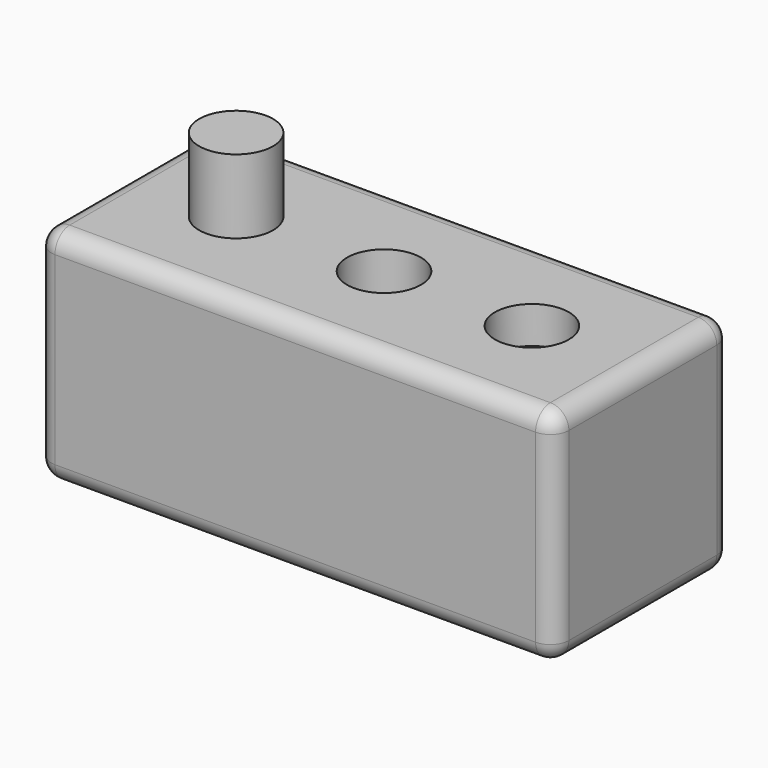
from build123d import *

# Parameters (mm, degrees)
F0_W          = 140
F0_H          = 60
F1_DEPTH      = 60
F2_R          = 10
F5_DEPTH      = 20
F4_R          = 10
F6_DEPTH      = 71.6
F3_R          = 10
F7_DEPTH      = 10
F8_R          = 5
F9_T1_DEPTH   = 165
F9_T3_DEPTH   = 67.5
F9_S7_W       = 5
F9_S7_H       = 5
F9_T8_DEPTH   = 5
F10_T1_DEPTH  = 50
F10_T3_DEPTH  = 67.5
F10_S7_W      = 5
F10_S7_H      = 5
F10_T8_DEPTH  = 5
F10_T12_ANGLE = 89.9999999974
F11_T1_DEPTH  = 147.5
F11_T3_DEPTH  = 50
F11_S7_W      = 5
F11_S7_H      = 5
F11_T8_DEPTH  = 5
F11_T12_ANGLE = 89.9999999974
F12_T1_DEPTH  = 50
F12_T3_DEPTH  = 50
F12_S7_W      = 5
F12_S7_H      = 5
F12_T8_DEPTH  = 5
F12_S13_W     = 5
F12_S13_H     = 5
F12_T14_DEPTH = 5
F12_T18_ANGLE = 89.9999999974


# Not quite as in the source:
# - a fillet or chamfer that OpenCascade refuses, or shapes differently, is made with other operations: its cross-section is extruded or revolved along the edge and cut away or added


with BuildPart() as f1:
    # F0 (on Top) → F1 (new body)
    with BuildSketch(Plane.XY):
        Rectangle(F0_W, F0_H)
    extrude(amount=F1_DEPTH)

    # F2 (on face) → F5 (join)
    with BuildSketch(Plane.XY.offset(60)):
        with Locations((-40, 0)):
            Circle(F2_R)
    extrude(amount=F5_DEPTH)

    # F4 (on face) → F6 (cut)
    with BuildSketch(Plane.XY.offset(60)):
        Circle(F4_R)
    extrude(amount=-F6_DEPTH, mode=Mode.SUBTRACT)

    # F3 (on face) → F7 (cut)
    with BuildSketch(Plane.XY.offset(60)):
        with Locations((40, 0)):
            Circle(F3_R)
    extrude(amount=-F7_DEPTH, mode=Mode.SUBTRACT)

    # F8
    f8_edges = [f1.edges().sort_by_distance(p)[0] for p in [
        (0, 30, 60),
        (-70, 0, 60),
        (0, -30, 60),
        (70, 0, 60),
    ]]
    fillet(f8_edges, radius=F8_R)

    # F9: fillet of radius 5 on 2 edges, made by hand

    # F9_s2 → F9_t1 (cut)
    with BuildSketch(Plane.YZ.offset(-82.5)):
        with BuildLine():
            ThreePointArc((-30, 5), (-28.5355339059, 1.4644660941), (-25, 0))
            Line((-25, 0), (-30, 0))
            Line((-30, 0), (-30, 5))
        make_face()
    extrude(amount=F9_T1_DEPTH, mode=Mode.SUBTRACT)

    # F9_s4 → F9_t3 (cut)
    with BuildSketch(Plane.XY.offset(-12.5)):
        with BuildLine():
            ThreePointArc((65, -30), (68.5355339059, -28.5355339059), (70, -25))
            Line((70, -25), (70, -30))
            Line((70, -30), (65, -30))
        make_face()
    extrude(amount=F9_T3_DEPTH, mode=Mode.SUBTRACT)


with BuildPart() as f9_tool6:
    # F9_s7 → F9_t8 (new body)
    with BuildSketch(Plane.XZ.offset(25)):
        with Locations((67.5, 57.5)):
            Rectangle(F9_S7_W, F9_S7_H)
    extrude(amount=F9_T8_DEPTH)

    # F9_s9 → F9_t10 (revolve, cut)
    with BuildSketch(Plane(origin=(65, -25, 55), x_dir=(-0.7071067812, 0, -0.7071067812), z_dir=(-0.7071067812, 0, 0.7071067812))):
        with BuildLine():
            ThreePointArc((0, -5), (5, 0), (0, 5))
            Line((0, 5), (0, -5))
        make_face()
    revolve(axis=Axis((65, -25, 55), (0, -1, 0)), mode=Mode.SUBTRACT)


with BuildPart() as f1_1:
    add(f1.part)

    # F9_t5: cut F9_tool6
    add(f9_tool6.part, mode=Mode.SUBTRACT)

    # F10: fillet of radius 5 on 1 edges, made by hand

    # F10_s2 → F10_t1 (cut)
    with BuildSketch(Plane.XY.offset(5)):
        with BuildLine():
            ThreePointArc((-65, -30), (-68.5355339059, -28.5355339059), (-70, -25))
            Line((-70, -25), (-70, -30))
            Line((-70, -30), (-65, -30))
        make_face()
    extrude(amount=F10_T1_DEPTH, mode=Mode.SUBTRACT)

    # F10_s4 → F10_t3 (cut)
    with BuildSketch(Plane.XZ.offset(-42.5)):
        with BuildLine():
            ThreePointArc((-70, 5), (-68.5355339059, 1.4644660941), (-65, 0))
            Line((-65, 0), (-70, 0))
            Line((-70, 0), (-70, 5))
        make_face()
    extrude(amount=F10_T3_DEPTH, mode=Mode.SUBTRACT)


with BuildPart() as f10_tool6:
    # F10_s7 → F10_t8 (new body)
    with BuildSketch(Plane.XZ.offset(25)):
        with Locations((-67.5, 57.5)):
            Rectangle(F10_S7_W, F10_S7_H)
    extrude(amount=F10_T8_DEPTH)

    # F10_s9 → F10_t10 (revolve, cut)
    with BuildSketch(Plane(origin=(-65, -25, 55), x_dir=(0.7071067812, 0, -0.7071067812), z_dir=(-0.7071067812, 0, -0.7071067812))):
        with BuildLine():
            ThreePointArc((0, -5), (5, 0), (0, 5))
            Line((0, 5), (0, -5))
        make_face()
    revolve(axis=Axis((-65, -25, 55), (0, -1, 0)), mode=Mode.SUBTRACT)


with BuildPart() as f1_2:
    add(f1_1.part)

    # F10_t5: cut F10_tool6
    add(f10_tool6.part, mode=Mode.SUBTRACT)

    # F10_s11 → F10_t12 (revolve, cut)
    with BuildSketch(Plane.XZ.offset(24.9999999999)):
        with BuildLine():
            ThreePointArc((-65, 0), (-68.5355339059, 1.4644660941), (-70, 5))
            Line((-70, 5), (-70, 0))
            Line((-70, 0), (-65, 0))
        make_face()
    revolve(axis=Axis((-70, -24.9999999999, 5.0000000001), (-1, 0, 0)), revolution_arc=F10_T12_ANGLE, mode=Mode.SUBTRACT)

    # F11: fillet of radius 5 on 1 edges, made by hand

    # F11_s2 → F11_t1 (cut)
    with BuildSketch(Plane.YZ.offset(-65)):
        with BuildLine():
            ThreePointArc((25, 0), (28.5355339059, 1.4644660941), (30, 5))
            Line((30, 5), (30, 0))
            Line((30, 0), (25, 0))
        make_face()
    extrude(amount=F11_T1_DEPTH, mode=Mode.SUBTRACT)

    # F11_s4 → F11_t3 (cut)
    with BuildSketch(Plane.XY.offset(5)):
        with BuildLine():
            ThreePointArc((-65, 30), (-68.5355339059, 28.5355339059), (-70, 25))
            Line((-70, 25), (-70, 30))
            Line((-70, 30), (-65, 30))
        make_face()
    extrude(amount=F11_T3_DEPTH, mode=Mode.SUBTRACT)


with BuildPart() as f11_tool6:
    # F11_s7 → F11_t8 (new body)
    with BuildSketch(Plane.XZ.offset(-25)):
        with Locations((-67.5, 57.5)):
            Rectangle(F11_S7_W, F11_S7_H)
    extrude(amount=-F11_T8_DEPTH)

    # F11_s9 → F11_t10 (revolve, cut)
    with BuildSketch(Plane(origin=(-65, 25, 55), x_dir=(0.7071067812, 0, -0.7071067812), z_dir=(0.7071067812, 0, 0.7071067812))):
        with BuildLine():
            ThreePointArc((0, -5), (5, 0), (0, 5))
            Line((0, 5), (0, -5))
        make_face()
    revolve(axis=Axis((-65, 25, 55), (0, 1, 0)), mode=Mode.SUBTRACT)


with BuildPart() as f1_3:
    add(f1_2.part)

    # F11_t5: cut F11_tool6
    add(f11_tool6.part, mode=Mode.SUBTRACT)

    # F11_s11 → F11_t12 (revolve, cut)
    with BuildSketch(Plane.YZ.offset(-64.9999999999)):
        with BuildLine():
            ThreePointArc((30, 5), (28.5355339059, 1.4644660941), (25, 0))
            Line((25, 0), (30, 0))
            Line((30, 0), (30, 5))
        make_face()
    revolve(axis=Axis((-64.9999999999, 30, 5.0000000001), (0, 1, 0)), revolution_arc=F11_T12_ANGLE, mode=Mode.SUBTRACT)

    # F12: fillet of radius 5 on 1 edges, made by hand

    # F12_s2 → F12_t1 (cut)
    with BuildSketch(Plane.XY.offset(5)):
        with BuildLine():
            ThreePointArc((70, 25), (68.5355339059, 28.5355339059), (65, 30))
            Line((65, 30), (70, 30))
            Line((70, 30), (70, 25))
        make_face()
    extrude(amount=F12_T1_DEPTH, mode=Mode.SUBTRACT)

    # F12_s4 → F12_t3 (cut)
    with BuildSketch(Plane.XZ.offset(-25)):
        with BuildLine():
            ThreePointArc((65, 0), (68.5355339059, 1.4644660941), (70, 5))
            Line((70, 5), (70, 0))
            Line((70, 0), (65, 0))
        make_face()
    extrude(amount=F12_T3_DEPTH, mode=Mode.SUBTRACT)


with BuildPart() as f12_tool6:
    # F12_s7 → F12_t8 (new body)
    with BuildSketch(Plane.YZ.offset(65)):
        with Locations((27.5, 57.5)):
            Rectangle(F12_S7_W, F12_S7_H)
    extrude(amount=F12_T8_DEPTH)

    # F12_s9 → F12_t10 (revolve, cut)
    with BuildSketch(Plane(origin=(65, 25, 55), x_dir=(0, -0.7071067812, -0.7071067812), z_dir=(0, -0.7071067812, 0.7071067812))):
        with BuildLine():
            ThreePointArc((0, -5), (5, 0), (0, 5))
            Line((0, 5), (0, -5))
        make_face()
    revolve(axis=Axis((65, 25, 55), (1, 0, 0)), mode=Mode.SUBTRACT)


with BuildPart() as f1_4:
    add(f1_3.part)

    # F12_t5: cut F12_tool6
    add(f12_tool6.part, mode=Mode.SUBTRACT)


with BuildPart() as f12_tool12:
    # F12_s13 → F12_t14 (new body)
    with BuildSketch(Plane.XY.offset(5)):
        with Locations((67.5, -27.5)):
            Rectangle(F12_S13_W, F12_S13_H)
    extrude(amount=-F12_T14_DEPTH)

    # F12_s15 → F12_t16 (revolve, cut)
    with BuildSketch(Plane(origin=(65, -25, 5), x_dir=(-0.7071067812, 0.7071067812, 0), z_dir=(-0.7071067812, -0.7071067812, 0))):
        with BuildLine():
            ThreePointArc((0, -5), (5, 0), (0, 5))
            Line((0, 5), (0, -5))
        make_face()
    revolve(axis=Axis((65, -25, 5), (0, 0, -1)), mode=Mode.SUBTRACT)


with BuildPart() as f1_5:
    add(f1_4.part)

    # F12_t11: cut F12_tool12
    add(f12_tool12.part, mode=Mode.SUBTRACT)

    # F12_s17 → F12_t18 (revolve, cut)
    with BuildSketch(Plane.XY.offset(5.0000000001)):
        with BuildLine():
            ThreePointArc((70, 25), (68.5355339059, 28.5355339059), (65, 30))
            Line((65, 30), (70, 30))
            Line((70, 30), (70, 25))
        make_face()
    revolve(axis=Axis((70, 24.9999999999, 5.0000000001), (-1, 0, 0)), revolution_arc=F12_T18_ANGLE, mode=Mode.SUBTRACT)


solid = f1_5.part
